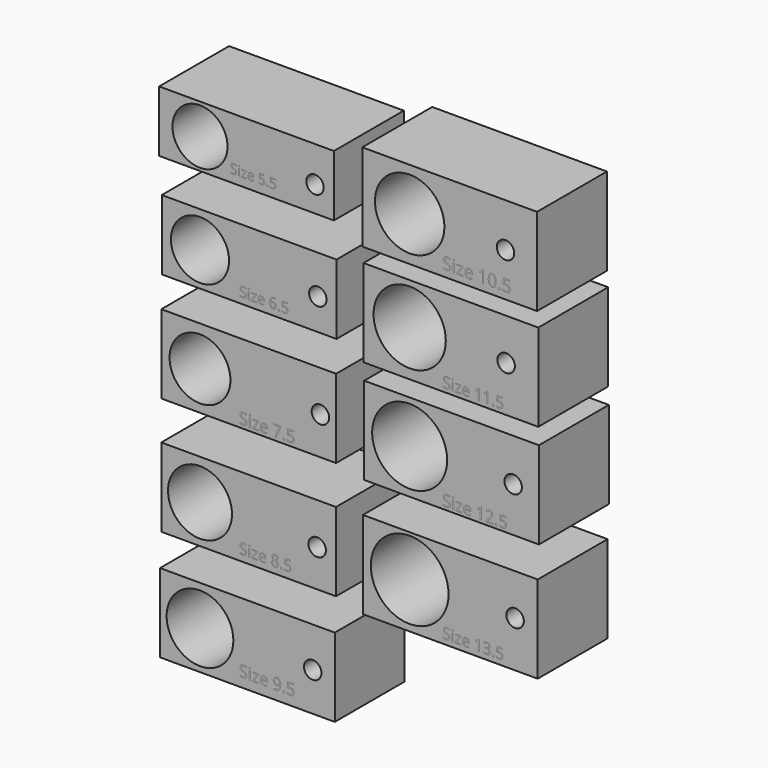
from build123d import *

# Parameters (mm, degrees)
F0_W           = 50.8
F0_H           = 17.78
F0_R           = 8
F0_R_2         = 2.54
F2_DEPTH       = 25.4
F0_H_2         = 20.32
F0_R_3         = 8.45
F0_H_3         = 22.86
F0_R_4         = 8.85
F0_R_5         = 9.3
F0_R_6         = 9.7
F0_H_4         = 25.4
F0_R_7         = 11.3
F0_R_8         = 10.9
F0_R_9         = 10.5
F0_R_10        = 10.1
F1_TEXT_SIZE   = 3.878849869
F1_TEXT_SIZE_2 = 4.1374393428
F1_TEXT_SIZE_3 = 4.6546182906
F1_TEXT_SIZE_4 = 4.3931882828
F1_TEXT_SIZE_5 = 4.6516044272
F1_TEXT_SIZE_6 = 4.9100360937
F1_TEXT_SIZE_7 = 4.3931934569
F1_TEXT_SIZE_8 = 4.6516134818
F3_DEPTH       = 25.4


# Not quite as in the source:
# - Text() gives the source's letters only with a copy of the font that has no kerning and outlines rounded to 1/6400 em; it was checked with that copy


with BuildPart() as f2:
    # F0 (on Front) → F2 (new body)
    with BuildSketch(Plane.XZ):
        with Locations((-43.6408870578, 59.5246784532)):
            Rectangle(F0_W, F0_H)
        with Locations((-57.1683645248, 59.45443362)):
            Circle(F0_R, mode=Mode.SUBTRACT)
        with Locations((-23.7361679643, 58.0499191263)):
            Circle(F0_R_2, mode=Mode.SUBTRACT)
    extrude(amount=F2_DEPTH)


with BuildPart() as f2b:
    # F0 (on Front) → F2, piece 2 (new body)
    with BuildSketch(Plane.XZ):
        with Locations((-42.8785212994, 30.7155651337)):
            Rectangle(F0_W, F0_H_2)
        with Locations((-57.1683645248, 30.4295811802)):
            Circle(F0_R_3, mode=Mode.SUBTRACT)
        with Locations((-22.9103676975, 29.6848434955)):
            Circle(F0_R_2, mode=Mode.SUBTRACT)
    extrude(amount=F2_DEPTH)


with BuildPart() as f2c:
    # F0 (on Front) → F2, piece 3 (new body)
    with BuildSketch(Plane.XZ):
        with Locations((-42.9995224535, 0.1843560471)):
            Rectangle(F0_W, F0_H_3)
        with Locations((-57.1683645248, 0)):
            Circle(F0_R_4, mode=Mode.SUBTRACT)
        with Locations((-22.1656281501, -0.2909031755)):
            Circle(F0_R_2, mode=Mode.SUBTRACT)
    extrude(amount=F2_DEPTH)


with BuildPart() as f2d:
    # F0 (on Front) → F2, piece 4 (new body)
    with BuildSketch(Plane.XZ):
        with Locations((-43.0261880815, -33.9212873501)):
            Rectangle(F0_W, F0_H_3)
        with Locations((-57.1683645248, -34.1765284538)):
            Circle(F0_R_5, mode=Mode.SUBTRACT)
        with Locations((-23.0965521187, -34.5488972962)):
            Circle(F0_R_2, mode=Mode.SUBTRACT)
    extrude(amount=F2_DEPTH)


with BuildPart() as f2e:
    # F0 (on Front) → F2, piece 5 (new body)
    with BuildSketch(Plane.XZ):
        with Locations((-43.3863640487, -66.1833891195)):
            Rectangle(F0_W, F0_H_3)
        with Locations((-57.1683645248, -66.3864910603)):
            Circle(F0_R_6, mode=Mode.SUBTRACT)
        with Locations((-24.3998467922, -66.3864910603)):
            Circle(F0_R_2, mode=Mode.SUBTRACT)
    extrude(amount=F2_DEPTH)


with BuildPart() as f2f:
    # F0 (on Front) → F2, piece 6 (new body)
    with BuildSketch(Plane.XZ):
        with Locations((15.6001312003, -34.6791970871)):
            Rectangle(F0_W, F0_H_4)
        with Locations((3.7841338199, -34.1765284538)):
            Circle(F0_R_7, mode=Mode.SUBTRACT)
        with Locations((34.4345346093, -33.99034217)):
            Circle(F0_R_2, mode=Mode.SUBTRACT)
    extrude(amount=F2_DEPTH)


with BuildPart() as f2g:
    # F0 (on Front) → F2, piece 7 (new body)
    with BuildSketch(Plane.XZ):
        with Locations((15.9687645078, -0.2048370291)):
            Rectangle(F0_W, F0_H_4)
        with Locations((3.7841338199, 0)):
            Circle(F0_R_8, mode=Mode.SUBTRACT)
        with Locations((33.8759869337, 0.081466329)):
            Circle(F0_R_2, mode=Mode.SUBTRACT)
    extrude(amount=F2_DEPTH)


with BuildPart() as f2h:
    # F0 (on Front) → F2, piece 8 (new body)
    with BuildSketch(Plane.XZ):
        with Locations((15.7760412708, 29.8450022608)):
            Rectangle(F0_W, F0_H_4)
        with Locations((3.7841338199, 30.4295811802)):
            Circle(F0_R_9, mode=Mode.SUBTRACT)
        with Locations((31.8279527128, 30.4295811802)):
            Circle(F0_R_2, mode=Mode.SUBTRACT)
    extrude(amount=F2_DEPTH)


with BuildPart() as f2i:
    # F0 (on Front) → F2, piece 9 (new body)
    with BuildSketch(Plane.XZ):
        with Locations((15.4120776147, 59.3417763382)):
            Rectangle(F0_W, F0_H_4)
        with Locations((3.7841338199, 59.45443362)):
            Circle(F0_R_10, mode=Mode.SUBTRACT)
        with Locations((31.6417664289, 59.2882148921)):
            Circle(F0_R_2, mode=Mode.SUBTRACT)
    extrude(amount=F2_DEPTH)


with BuildPart() as f3:
    # F1 (on Front) → F3 (new body)
    with BuildSketch(Plane.XZ):
        with Locations((-48.4176799655, 52.9579371214)):
            Text('Size 5.5', F1_TEXT_SIZE, font='Open Sans', text_align=(TextAlign.LEFT, TextAlign.BOTTOM))
        with Locations((-45.8110943437, 22.2374517471)):
            Text('Size 6.5', F1_TEXT_SIZE_2, font='Open Sans', text_align=(TextAlign.LEFT, TextAlign.BOTTOM))
        with Locations((-45.8110943437, -10.3448797017)):
            Text('Size 7.5', F1_TEXT_SIZE_3, font='Open Sans', text_align=(TextAlign.LEFT, TextAlign.BOTTOM))
        with Locations((-45.8110943437, -43.5945801437)):
            Text('Size 8.5', F1_TEXT_SIZE_4, font='Open Sans', text_align=(TextAlign.LEFT, TextAlign.BOTTOM))
        with Locations((-45.8110943437, -75.0394910574)):
            Text('Size 9.5', F1_TEXT_SIZE_5, font='Open Sans', text_align=(TextAlign.LEFT, TextAlign.BOTTOM))
        with Locations((13.3036179468, 48.5073886812)):
            Text('Size 10.5', F1_TEXT_SIZE_6, font='Open Sans', text_align=(TextAlign.LEFT, TextAlign.BOTTOM))
        with Locations((13.3036179468, 18.1788615882)):
            Text('Size 11.5', F1_TEXT_SIZE_7, font='Open Sans', text_align=(TextAlign.LEFT, TextAlign.BOTTOM))
        with Locations((13.3036179468, -12.1496655047)):
            Text('Size 12.5', F1_TEXT_SIZE_8, font='Open Sans', text_align=(TextAlign.LEFT, TextAlign.BOTTOM))
        with Locations((13.3036179468, -46.0134185851)):
            Text('Size 13.5', F1_TEXT_SIZE_4, font='Open Sans', text_align=(TextAlign.LEFT, TextAlign.BOTTOM))
    extrude(amount=F3_DEPTH)


solid = Compound([f2.part, f2b.part, f2c.part, f2d.part, f2e.part, f2f.part, f2g.part, f2h.part, f2i.part, f3.part])
